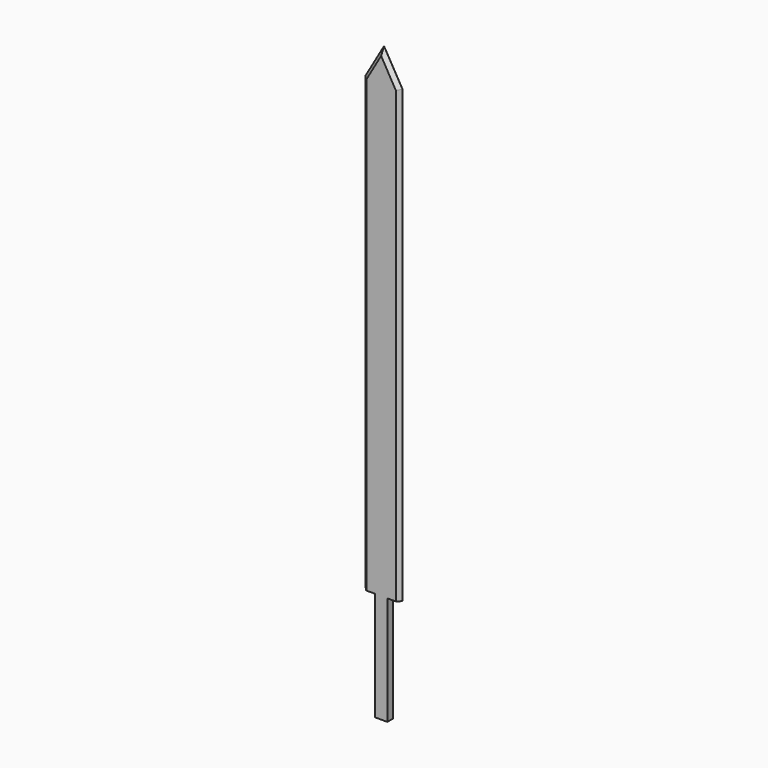
from build123d import *

# Parameters (mm, degrees)
F0_W        = 2.6332533453
F0_H        = 23.0305567384
F1_DEPTH    = 1.524
F2_SIZE     = 1
F3_SIZE     = 1
F4_T1_DEPTH = 13.8806275065
F5_T1_DEPTH = 12.7259269681
F6_SIZE     = 1
F7_T1_DEPTH = 98.6181021709
F8_SIZE     = 1
F9_T1_DEPTH = 98.6181021709


# Not quite as in the source:
# - a fillet or chamfer that OpenCascade refuses, or shapes differently, is made with other operations: its cross-section is extruded or revolved along the edge and cut away or added


with BuildPart() as f1:
    # F0 (on Front) → F1 (new body)
    with BuildSketch(Plane.XZ):
        Polygon((-4.1333585978, 47.5307323504), (4.1333585978, 47.5307323504), (4.3686307653, 47.5307323504), (0, 55.0974227954), (-4.3686307653, 47.5307323504), align=None)
        Polygon((4.1333585978, -47.5365004968), (4.1333585978, 47.5307323504), (-4.1333585978, 47.5307323504), (-4.1333585978, -47.5365004968), (-1.3166266726, -47.5365004968), (1.3166266726, -47.5365004968), align=None)
        with Locations((0, -59.051778866)):
            Rectangle(F0_W, F0_H)
    extrude(amount=F1_DEPTH)

    # F2
    f2_edges = [f1.edges().sort_by_distance(p)[0] for p in [
        (-2.184315, -1.524, 51.314078),
    ]]
    chamfer(f2_edges, length=F2_SIZE)

    # F3
    f3_edges = [f1.edges().sort_by_distance(p)[0] for p in [
        (2.472991, -1.524, 50.814078),
    ]]
    chamfer(f3_edges, length=F3_SIZE)

    # F4: chamfer of 1 on 1 edges, made by hand

    # F4_s2 → F4_t1 (cut)
    with BuildSketch(Plane(origin=(-18.2034116527, 0, 31.5292338535), x_dir=(0, 1, 0), z_dir=(-0.5, 0, 0.8660254038))):
        Polygon((-1, -27.5487113977), (0, -26.5487113977), (0, -27.5487113977), align=None)
    extrude(amount=F4_T1_DEPTH, mode=Mode.SUBTRACT)

    # F5: chamfer of 1 on 1 edges, made by hand

    # F5_s2 → F5_t1 (cut)
    with BuildSketch(Plane(origin=(24.5663751367, 0, 42.5502098946), x_dir=(0, 1, 0), z_dir=(-0.5, 0, -0.8660254038))):
        Polygon((0, -26.5487113977), (-1, -27.5487113977), (0, -27.5487113977), align=None)
    extrude(amount=F5_T1_DEPTH, mode=Mode.SUBTRACT)

    # F6
    f6_edges = [f1.edges().sort_by_distance(p)[0] for p in [
        (4.133359, -1.524, -0.799132),
    ]]
    chamfer(f6_edges, length=F6_SIZE)

    # F7: chamfer of 1 on 1 edges, made by hand

    # F7_s2 → F7_t1 (cut)
    with BuildSketch(Plane.XY.offset(-50.1081834848)):
        Polygon((4.1333585978, -1), (3.1333585978, 0), (4.1333585978, 0), align=None)
    extrude(amount=F7_T1_DEPTH, mode=Mode.SUBTRACT)

    # F8
    f8_edges = [f1.edges().sort_by_distance(p)[0] for p in [
        (-4.133359, 0, -0.799132),
    ]]
    chamfer(f8_edges, length=F8_SIZE)

    # F9: chamfer of 1 on 1 edges, made by hand

    # F9_s2 → F9_t1 (cut)
    with BuildSketch(Plane.XY.offset(-50.1081834848)):
        Polygon((-4.1333585978, -0.524), (-3.1333585978, -1.524), (-4.1333585978, -1.524), align=None)
    extrude(amount=F9_T1_DEPTH, mode=Mode.SUBTRACT)


solid = f1.part
